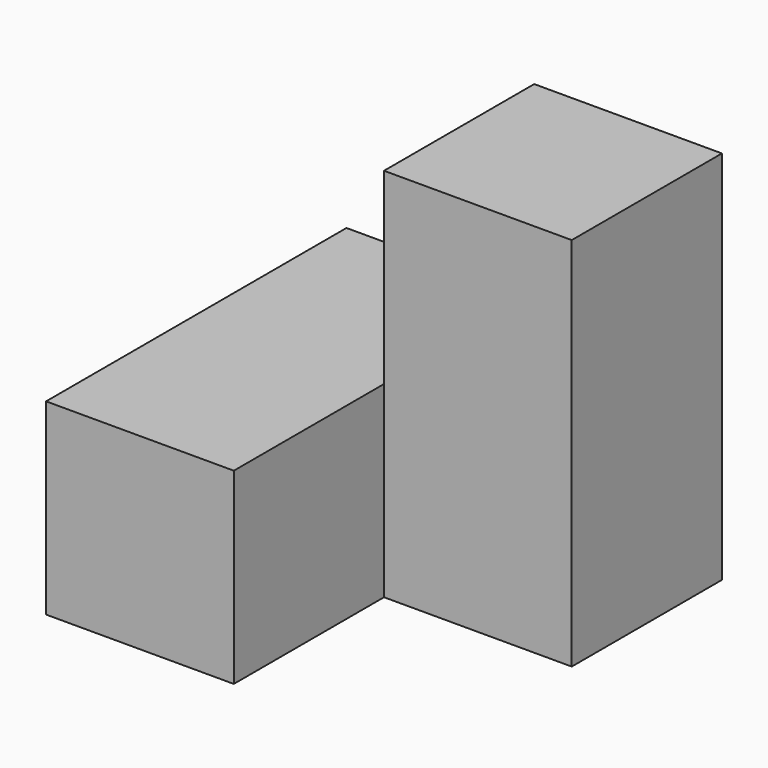
from build123d import *

# Parameters (mm, degrees)
F1_W     = 127
F1_H     = 127
F2_DEPTH = 127
F3_W     = 127
F3_H     = 127
F4_DEPTH = 127
F5_W     = 127
F5_H     = 127
F6_DEPTH = 127


# Not quite as in the source:
# - a variable given as a bare number and used for a length is read in inches; the dataset says mm whatever the document's units were


with BuildPart() as f2:
    # F1 (on Front) → F2 (new body, symmetric)
    with BuildSketch(Plane.XZ):
        Rectangle(F1_W, F1_H)
    extrude(amount=F2_DEPTH, both=True)

    # F3 (on face) → F4 (join)
    with BuildSketch(Plane.YZ.offset(63.5)):
        with Locations((63.5, 0)):
            Rectangle(F3_W, F3_H)
    extrude(amount=F4_DEPTH)

    # F5 (on face) → F6 (join)
    with BuildSketch(Plane.XY.offset(63.5)):
        with Locations((127, 63.5)):
            Rectangle(F5_W, F5_H)
    extrude(amount=F6_DEPTH)


solid = f2.part
